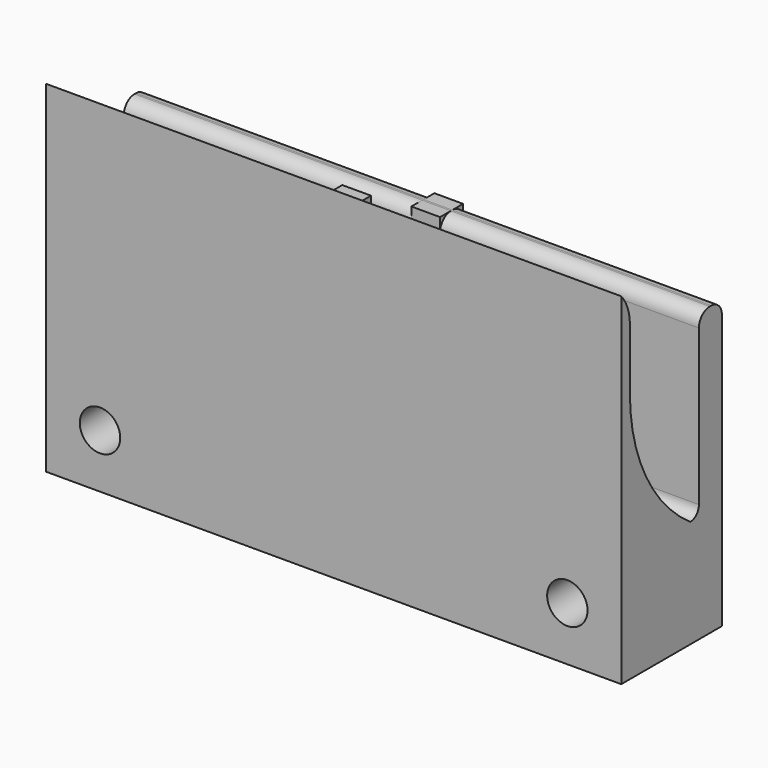
from build123d import *

# Parameters (mm, degrees)
F1_DEPTH       = 3.2
F2_DEPTH       = 32
F4_DEPTH       = 38.001
F5_R           = 6
F6_DEPTH       = 3.2
F7_SIZE        = 2
F8_T1_DEPTH    = 71.5
F9_D           = 4.4958
F9_CSINK_D     = 9.1186
F9_CSINK_ANGLE = 82
F10_T1_DEPTH   = 80.2480768093


# Not quite as in the source:
# - a fillet or chamfer that OpenCascade refuses, or shapes differently, is made with other operations: its cross-section is extruded or revolved along the edge and cut away or added


with BuildPart() as f1:
    # F0 (on Right) → F1 (new body)
    with BuildSketch(Plane.YZ):
        with BuildLine():
            Line((1.2, 28), (1.2, 38))
            Line((1.2, 38), (0, 38))
            Line((0, 38), (0, 0))
            Line((0, 0), (14, 0))
            Line((14, 0), (14, 32))
            Line((14, 32), (10.8, 32))
            Line((10.8, 32), (10.8, 13.2))
            ThreePointArc((10.8, 13.2), (10.4485281374, 12.3514718626), (9.6, 12))
            ThreePointArc((9.6, 12), (3.4276464791, 18.9645144015), (1.2, 28))
        make_face()
    extrude(amount=F1_DEPTH)


with BuildPart() as f2:
    # F0 (on Right) → F2 (new body, symmetric)
    with BuildSketch(Plane.YZ):
        with BuildLine():
            Line((1.2, 28), (1.2, 38))
            Line((1.2, 38), (0, 38))
            Line((0, 38), (0, 0))
            Line((0, 0), (14, 0))
            Line((14, 0), (14, 32))
            Line((14, 32), (10.8, 32))
            Line((10.8, 32), (10.8, 13.2))
            ThreePointArc((10.8, 13.2), (10.4485281374, 12.3514718626), (9.6, 12))
            ThreePointArc((9.6, 12), (3.4276464791, 18.9645144015), (1.2, 28))
        make_face()
    extrude(amount=F2_DEPTH, both=True)

    # F3 (on Top) → F4 (cut, through all)
    with BuildSketch(Plane.XY):
        with BuildLine():
            ThreePointArc((13.15, 7.3), (12.1395183951, 9.7395183951), (9.7, 10.75))
            Line((9.7, 10.75), (-9.7, 10.75))
            ThreePointArc((-9.7, 10.75), (-12.1395183951, 9.7395183951), (-13.15, 7.3))
            ThreePointArc((-13.15, 7.3), (-12.1395183951, 4.8604816049), (-9.7, 3.85))
            Line((-9.7, 3.85), (9.7, 3.85))
            ThreePointArc((9.7, 3.85), (12.1395183951, 4.8604816049), (13.15, 7.3))
        make_face()
    extrude(amount=F4_DEPTH, mode=Mode.SUBTRACT)

    # F5 (on face) → F6 (cut, through all)
    with BuildSketch(Plane(origin=(0, 14, 0), x_dir=(-1, 0, 0), z_dir=(0, 1, 0))):
        with Locations((0, 22.8)):
            Circle(F5_R)
    extrude(amount=-F6_DEPTH, mode=Mode.SUBTRACT)

    # F7
    f7_edges = [f2.edges().sort_by_distance(p)[0] for p in [
        (6, 14, 22.8),
    ]]
    chamfer(f7_edges, length=F7_SIZE)

    # F8: fillet of radius 1.5 on 2 edges, made by hand

    # F8_s2 → F8_t1 (cut)
    with BuildSketch(Plane.YZ.offset(-35.75)):
        with BuildLine():
            ThreePointArc((14, 30.5), (13.5606601718, 31.5606601718), (12.5, 32))
            Line((12.5, 32), (14, 32))
            Line((14, 32), (14, 30.5))
        make_face()
        with BuildLine():
            ThreePointArc((12.3, 32), (11.2393398282, 31.5606601718), (10.8, 30.5))
            Line((10.8, 30.5), (10.8, 32))
            Line((10.8, 32), (12.3, 32))
        make_face()
    extrude(amount=F8_T1_DEPTH, mode=Mode.SUBTRACT)

    # F9 (through all)
    with Locations(Plane(origin=(0, 14, 0), x_dir=(-1, 0, 0), z_dir=(0, 1, 0))):
        with Locations((-26, 6), (26, 6)):
            CounterSinkHole(F9_D / 2, F9_CSINK_D / 2, counter_sink_angle=F9_CSINK_ANGLE)

    # F10: fillet of radius 5 on 1 edges, made by hand

    # F10_s2 → F10_t1 (cut)
    with BuildSketch(Plane.YZ.offset(-40.1240384046)):
        with BuildLine():
            ThreePointArc((0, 38), (0.8904157598, 36.4824354457), (1.2, 34.7503846381))
            Line((1.2, 34.7503846381), (1.2, 38))
            Line((1.2, 38), (0, 38))
        make_face()
    extrude(amount=F10_T1_DEPTH, mode=Mode.SUBTRACT)


solid = Compound([f1.part, f2.part])
